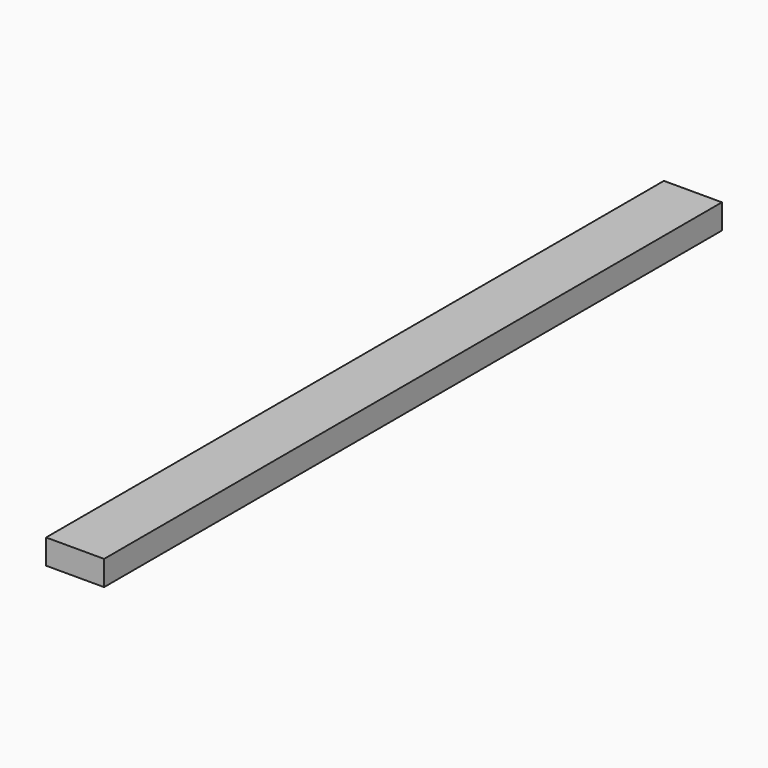
from build123d import *

# Parameters (mm, degrees)
F1_W     = 88.9
F1_H     = 38.1
F2_DEPTH = 1183.132


# Not quite as in the source:
# - a variable given as a bare number and used for a length is read in inches; the dataset says mm whatever the document's units were


with BuildPart() as f2:
    # F1 (on Front) → F2 (new body)
    with BuildSketch(Plane.XZ):
        Rectangle(F1_W, F1_H)
    extrude(amount=F2_DEPTH)


solid = f2.part
